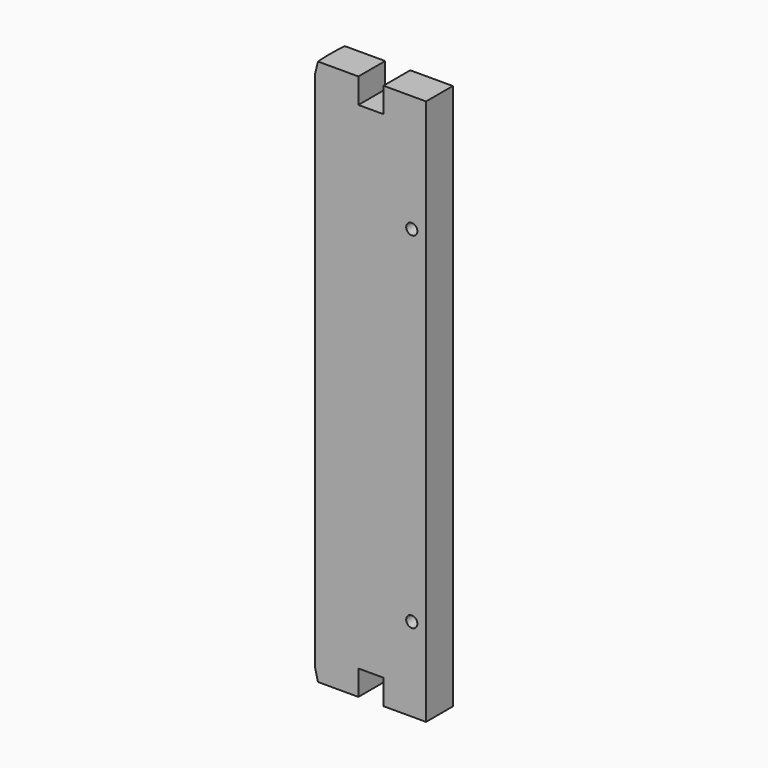
from build123d import *

# Parameters (mm, degrees)
F0_W        = 127
F0_H        = 622.3
F1_DEPTH    = 19.05
F3_DEPTH    = 622.301
F5_D        = 12.7
F6_W        = 28.575
F6_H        = 28.575
F7_DEPTH    = 38.101
F8_C1_SIZE2 = 12.7
F8_C1_SIZE  = 3.175
F8_C2_SIZE2 = 3.175
F8_C2_SIZE  = 12.7


# Not quite as in the source:
# - a length typed as a fraction of an inch, garbled in the dataset ("3 / 203.2 mm" for 3/8 in), is restored
# - a pattern or mirror of a feature is missing from the dataset's text; its kind, count and spacing are read off the source's solid


with BuildPart() as f1:
    # F0 (on Front) → F1 (new body, symmetric)
    with BuildSketch(Plane.XZ):
        Rectangle(F0_W, F0_H)
    extrude(amount=F1_DEPTH, both=True)

    # F2 (on face) → F3 (cut, through all)
    with BuildSketch(Plane.XY.offset(311.15)):
        with BuildLine():
            ThreePointArc((-63.5, 2.159e-07), (-63.3181995898, 9.5319324627), (-62.773062814, 19.05))
            Line((-62.773062814, 19.05), (-63.5, 19.05))
            Line((-63.5, 19.05), (-63.5, 2.159e-07))
        make_face()
        with BuildLine():
            Line((-63.5, -19.05), (-62.773062814, -19.05))
            ThreePointArc((-62.773062814, -19.05), (-63.318199598, -9.531932247), (-63.5, 2.159e-07))
            Line((-63.5, 2.159e-07), (-63.5, -19.05))
        make_face()
    extrude(amount=-F3_DEPTH, mode=Mode.SUBTRACT)

    # F5 (through all)
    with Locations(Plane.XZ.offset(19.05)):
        with Locations((47.244, 177.8), (47.244, -215.9)):
            Hole(F5_D / 2)

    # F6 (on face) → F7 (cut, through all)
    with BuildSketch(Plane.XZ.offset(19.05)):
        with Locations((0.7239, 296.8625)):
            Rectangle(F6_W, F6_H)
    f7 = extrude(amount=-F7_DEPTH, mode=Mode.SUBTRACT)

    # F7_copies: F7 across plane
    add(f7.mirror(Plane(origin=(0, 0, 0), x_dir=(-1, 0, 0), z_dir=(0, 0, -1))), mode=Mode.SUBTRACT)

    # F8: chamfer of 12.7 x 3.175 on 2 edges, made by hand

    # F8_c1
    f8_c1_edges = [f1.edges().sort_by_distance(p)[0] for p in [
        (-63.5, 0, -311.15),
    ]]
    f8_c1_side = f1.faces().sort_by_distance((-63.4365, 0, -311.15))[0]
    chamfer(f8_c1_edges, length=F8_C1_SIZE, length2=F8_C1_SIZE2, reference=f8_c1_side)

    # F8_c2
    f8_c2_edges = [f1.edges().sort_by_distance(p)[0] for p in [
        (-63.5, 0, 311.15),
    ]]
    f8_c2_side = f1.faces().sort_by_distance((-63.5, 0, 311.0865))[0]
    chamfer(f8_c2_edges, length=F8_C2_SIZE, length2=F8_C2_SIZE2, reference=f8_c2_side)


solid = f1.part
